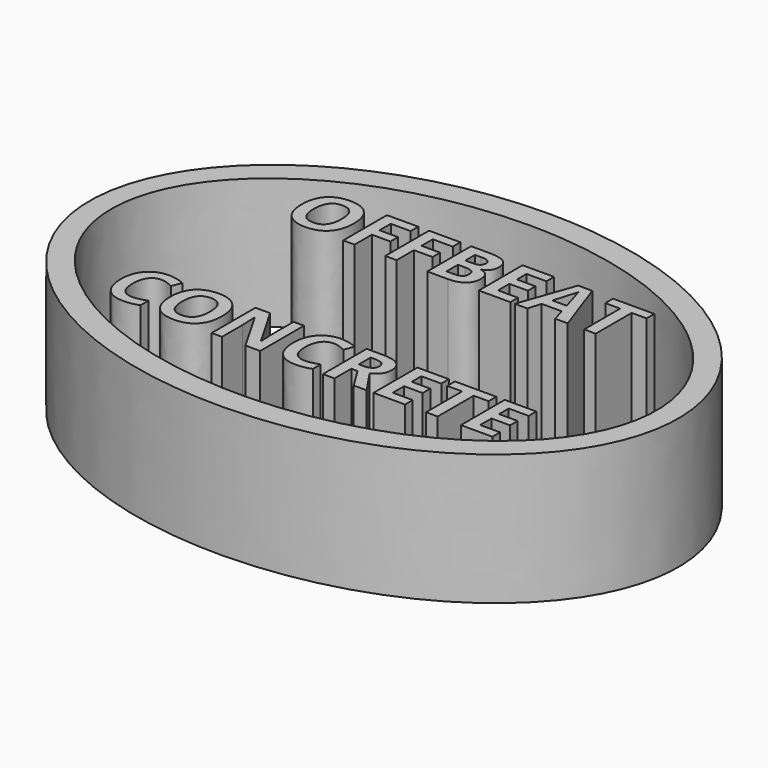
from build123d import *

# Parameters (mm, degrees)
F3_DEPTH       = 19.05
F1_TEXT_SIZE   = 11.153114287
F1_TEXT_SIZE_2 = 11.1680296767
F4_DEPTH       = 19.05


# Not quite as in the source:
# - Text() gives the source's letters only with a copy of the font that has no kerning and outlines rounded to 1/6400 em; it was checked with that copy


with BuildPart() as f3:
    # F0 (on Top) → F3 (new body)
    with BuildSketch(Plane.XY):
        with BuildLine():
            add(Edge.make_bspline(
                [(0, 30.1625), (-74.2400277394, 30.1625), (-37.1200138697, -15.08125), (0, -60.325), (37.1200138697, -15.08125), (74.2400277394, 30.1625), (0, 30.1625)],
                knots=[4.7123889804, 4.7123889804, 4.7123889804, 6.8067840828, 6.8067840828, 8.9011791852, 8.9011791852, 10.9955742876, 10.9955742876, 10.9955742876], degree=2, weights=[1, 0.5, 1, 0.5, 1, 0.5, 1]))
        make_face()
        with BuildLine():
            add(Edge.make_bspline(
                [(0, 26.551383851), (-68.7407664254, 26.551383851), (-34.3703832127, -13.2756919255), (0, -53.102767702), (34.3703832127, -13.2756919255), (68.7407664254, 26.551383851), (0, 26.551383851)],
                knots=[4.7123889804, 4.7123889804, 4.7123889804, 6.8067840828, 6.8067840828, 8.9011791852, 8.9011791852, 10.9955742876, 10.9955742876, 10.9955742876], degree=2, weights=[1, 0.5, 1, 0.5, 1, 0.5, 1]))
        make_face(mode=Mode.SUBTRACT)
    extrude(amount=F3_DEPTH)


with BuildPart() as f4:
    # F1 (on Top) → F4 (new body)
    with BuildSketch(Plane.XY):
        with Locations((-24.1469908506, 10.4113752022)):
            Text('OFFBEAT', F1_TEXT_SIZE, font='Open Sans', font_style=FontStyle.BOLD, text_align=(TextAlign.LEFT, TextAlign.BOTTOM))
        with Locations((-28.7134276405, -16.7339043692)):
            Text('CONCRETE', F1_TEXT_SIZE_2, font='Open Sans', font_style=FontStyle.BOLD, text_align=(TextAlign.LEFT, TextAlign.BOTTOM))
    extrude(amount=F4_DEPTH)


solid = Compound([f3.part, f4.part])
